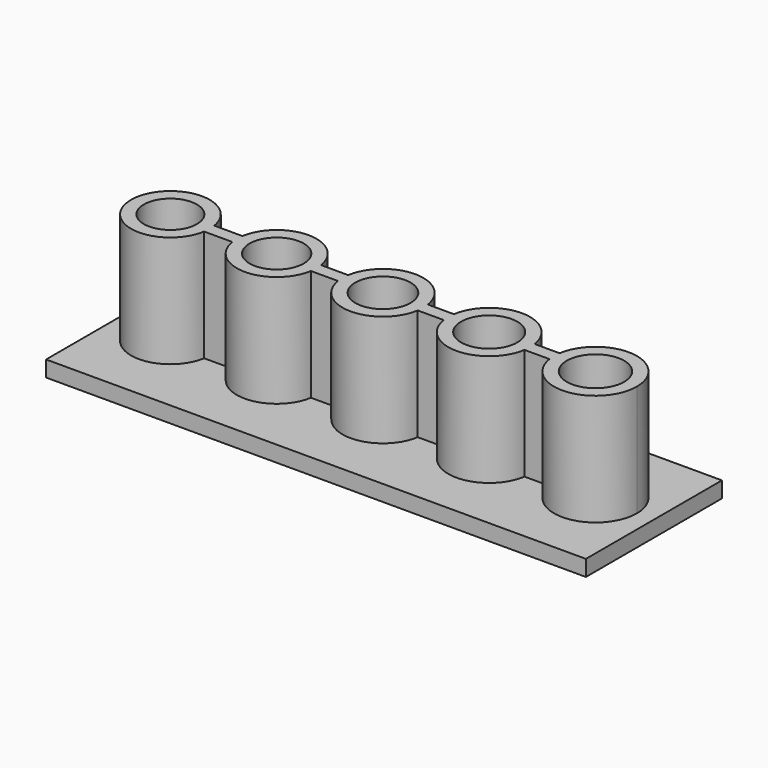
from build123d import *

# Parameters (mm, degrees)
F1_DEPTH = 1.5
F0_R     = 2.5
F0_R_2   = 2.55
F0_R_3   = 2.6
F0_R_4   = 2.65
F0_R_5   = 2.7
F2_DEPTH = 12


# Not quite as in the source:
# - a feature names something its author has since deleted; it is built from what else it names


with BuildPart() as f1:
    # F0 (on Top) → F1 (new body)
    with BuildSketch(Plane.XY):
        Polygon((-25.3, 5.5549060926), (-25.3, -8), (25.5, -8), (25.5, 8), (-22.4224738777, 8), (-22.4224738777, 5.5549060926), align=None)
        with BuildLine():
            ThreePointArc((-16.3489727473, -0.6), (-23.7, 0), (-16.3489727473, 0.6))
            Line((-16.3489727473, 0.6), (-13.7016888038, 0.6))
            ThreePointArc((-13.7016888038, 0.6), (-10, 3.75), (-6.2983111962, 0.6))
            Line((-6.2983111962, 0.6), (-3.7523326079, 0.6))
            ThreePointArc((-3.7523326079, 0.6), (0, 3.8), (3.7523326079, 0.6))
            Line((3.7523326079, 0.6), (6.197040626, 0.6))
            ThreePointArc((6.197040626, 0.6), (10, 3.85), (13.802959374, 0.6))
            Line((13.802959374, 0.6), (16.1464302264, 0.6))
            ThreePointArc((16.1464302264, 0.6), (20.3008968951, 3.888375118), (23.9, 0))
            ThreePointArc((23.9, 0), (20.3008968951, -3.888375118), (16.1464302264, -0.6))
            Line((16.1464302264, -0.6), (13.802959374, -0.6))
            ThreePointArc((13.802959374, -0.6), (10, -3.85), (6.197040626, -0.6))
            Line((6.197040626, -0.6), (3.7523326079, -0.6))
            ThreePointArc((3.7523326079, -0.6), (0, -3.8), (-3.7523326079, -0.6))
            Line((-3.7523326079, -0.6), (-6.2983111962, -0.6))
            ThreePointArc((-6.2983111962, -0.6), (-10, -3.75), (-13.7016888038, -0.6))
            Line((-13.7016888038, -0.6), (-16.3489727473, -0.6))
        make_face(mode=Mode.SUBTRACT)
    extrude(amount=F1_DEPTH)

    # F0 (on Top) → F2 (join)
    with BuildSketch(Plane.XY):
        with BuildLine():
            ThreePointArc((-16.3489727473, -0.6), (-16.3122635103, -0.3009976453), (-16.3, 0))
            ThreePointArc((-16.3, 0), (-16.3122635103, 0.3009976453), (-16.3489727473, 0.6))
            ThreePointArc((-16.3489727473, 0.6), (-23.7, 0), (-16.3489727473, -0.6))
        make_face()
        with Locations((-20, 0)):
            Circle(F0_R, mode=Mode.SUBTRACT)
        with BuildLine():
            ThreePointArc((-16.3489727473, 0.6), (-16.3122635103, 0.3009976453), (-16.3, 0))
            ThreePointArc((-16.3, 0), (-16.3122635103, -0.3009976453), (-16.3489727473, -0.6))
            Line((-16.3489727473, -0.6), (-13.7016888038, -0.6))
            ThreePointArc((-13.7016888038, -0.6), (-13.75, 0), (-13.7016888038, 0.6))
            Line((-13.7016888038, 0.6), (-16.3489727473, 0.6))
        make_face()
        with BuildLine():
            ThreePointArc((-6.2983111962, 0.6), (-10, 3.75), (-13.7016888038, 0.6))
            ThreePointArc((-13.7016888038, 0.6), (-13.75, 0), (-13.7016888038, -0.6))
            ThreePointArc((-13.7016888038, -0.6), (-10, -3.75), (-6.2983111962, -0.6))
            ThreePointArc((-6.2983111962, -0.6), (-6.2620973117, -0.3009709171), (-6.25, 0))
            ThreePointArc((-6.25, 0), (-6.2620973117, 0.3009709171), (-6.2983111962, 0.6))
        make_face()
        with Locations((-10, 0)):
            Circle(F0_R_2, mode=Mode.SUBTRACT)
        with BuildLine():
            Line((-3.7523326079, 0.6), (-6.2983111962, 0.6))
            ThreePointArc((-6.2983111962, 0.6), (-6.2620973117, 0.3009709171), (-6.25, 0))
            ThreePointArc((-6.25, 0), (-6.2620973117, -0.3009709171), (-6.2983111962, -0.6))
            Line((-6.2983111962, -0.6), (-3.7523326079, -0.6))
            ThreePointArc((-3.7523326079, -0.6), (-3.8, 0), (-3.7523326079, 0.6))
        make_face()
        with BuildLine():
            ThreePointArc((3.7523326079, 0.6), (0, 3.8), (-3.7523326079, 0.6))
            ThreePointArc((-3.7523326079, 0.6), (-3.8, 0), (-3.7523326079, -0.6))
            ThreePointArc((-3.7523326079, -0.6), (0, -3.8), (3.7523326079, -0.6))
            ThreePointArc((3.7523326079, -0.6), (3.7880644074, -0.3009452526), (3.8, 0))
            ThreePointArc((3.8, 0), (3.7880644074, 0.3009452526), (3.7523326079, 0.6))
        make_face()
        Circle(F0_R_3, mode=Mode.SUBTRACT)
        with BuildLine():
            Line((6.197040626, 0.6), (3.7523326079, 0.6))
            ThreePointArc((3.7523326079, 0.6), (3.7880644074, 0.3009452526), (3.8, 0))
            ThreePointArc((3.8, 0), (3.7880644074, -0.3009452526), (3.7523326079, -0.6))
            Line((3.7523326079, -0.6), (6.197040626, -0.6))
            ThreePointArc((6.197040626, -0.6), (6.15, 0), (6.197040626, 0.6))
        make_face()
        with BuildLine():
            ThreePointArc((13.802959374, 0.6), (10, 3.85), (6.197040626, 0.6))
            ThreePointArc((6.197040626, 0.6), (6.15, 0), (6.197040626, -0.6))
            ThreePointArc((6.197040626, -0.6), (10, -3.85), (13.802959374, -0.6))
            ThreePointArc((13.802959374, -0.6), (13.8382218272, -0.300920596), (13.85, 0))
            ThreePointArc((13.85, 0), (13.8382218272, 0.300920596), (13.802959374, 0.6))
        make_face()
        with Locations((10, 0)):
            Circle(F0_R_4, mode=Mode.SUBTRACT)
        with BuildLine():
            Line((16.1464302264, 0.6), (13.802959374, 0.6))
            ThreePointArc((13.802959374, 0.6), (13.8382218272, 0.300920596), (13.85, 0))
            ThreePointArc((13.85, 0), (13.8382218272, -0.300920596), (13.802959374, -0.6))
            Line((13.802959374, -0.6), (16.1464302264, -0.6))
            ThreePointArc((16.1464302264, -0.6), (16.1, 0), (16.1464302264, 0.6))
        make_face()
        with BuildLine():
            ThreePointArc((23.9, 0), (20.3008968951, 3.888375118), (16.1464302264, 0.6))
            ThreePointArc((16.1464302264, 0.6), (16.1, 0), (16.1464302264, -0.6))
            ThreePointArc((16.1464302264, -0.6), (20.3008968951, -3.888375118), (23.9, 0))
        make_face()
        with Locations((20, 0)):
            Circle(F0_R_5, mode=Mode.SUBTRACT)
    extrude(amount=F2_DEPTH)


solid = f1.part
